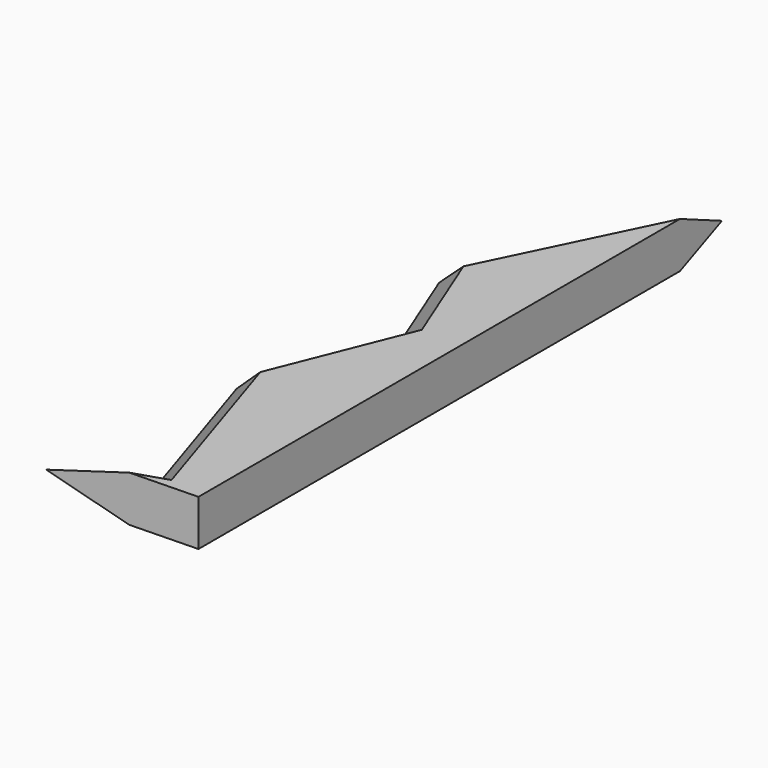
from build123d import *

# Parameters (mm, degrees)
F1_DEPTH = 5.08
F2_SIZE  = 2.53999


# Not quite as in the source:
# - a fillet or chamfer is up to 0.001 mm smaller than in the source, because OpenCascade refuses the exact size


with BuildPart() as f1:
    # F0 (on Top) → F1 (new body)
    with BuildSketch(Plane.XY):
        Polygon((0, 0), (0, 72.3038464785), (-11.8312668055, 48.0264090002), (-7.1868877858, 36.4154614508), (-13.0979157984, 21.6378867626), (-6.9757793099, 2.6381509379), (-16.4937096578, -0.428737424), align=None)
    extrude(amount=F1_DEPTH)

    # F2 (size 2.54 in the source; OpenCascade refuses exactly that, so slightly less here)
    f2_edges = [f1.edges().sort_by_distance(p)[0] for p in [
        (-5.915633, 60.165128, 5.08),
        (-9.509077, 42.220935, 5.08),
        (-10.142402, 29.026674, 5.08),
        (-10.036848, 12.138019, 5.08),
        (-11.734744, 1.104707, 5.08),
        (-5.915633, 60.165128, 0),
        (-9.509077, 42.220935, 0),
        (-10.142402, 29.026674, 0),
        (-10.036848, 12.138019, 0),
        (-11.734744, 1.104707, 0),
    ]]
    chamfer(f2_edges, length=F2_SIZE)


solid = f1.part
